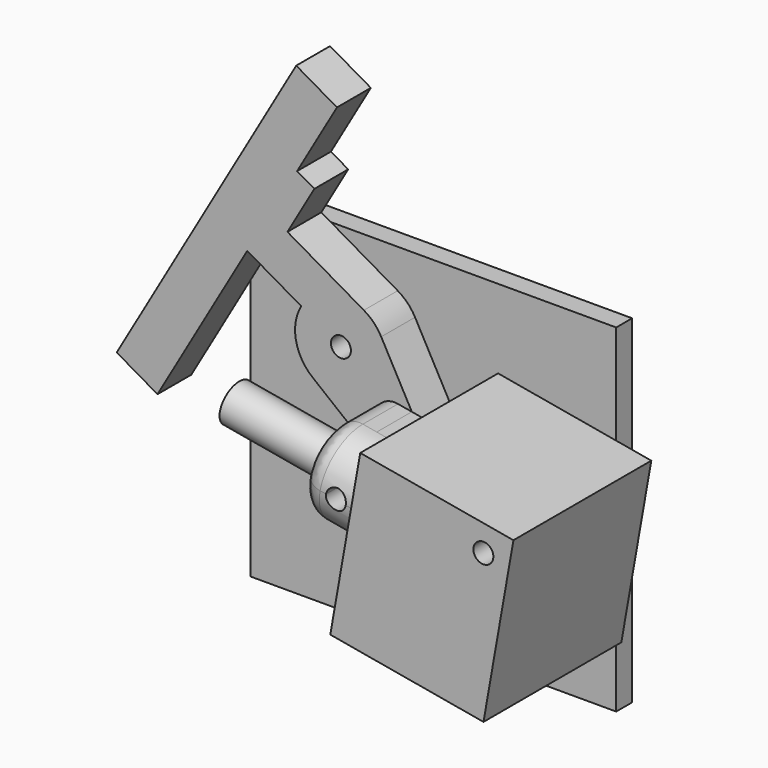
from build123d import *

# Parameters (mm, degrees)
F1_DEPTH    = 10.6
F2_DEPTH    = 43.2
F3_R        = 11
F4_DEPTH    = 2
F5_R        = 5
F6_DEPTH    = 43.4
F8_DEPTH    = 22
F9_T1_DEPTH = 73
F9_T3_DEPTH = 73
F10_W       = 91.6676837951
F10_H       = 84.7782492638
F11_DEPTH   = 5
F12_R       = 2.5
F13_DEPTH   = 74.8
F15_DEPTH   = 10.6
F16_R       = 5


# Not quite as in the source:
# - a fillet or chamfer that OpenCascade refuses, or shapes differently, is made with other operations: its cross-section is extruded or revolved along the edge and cut away or added
# - a feature names something its author has since deleted; it is built from what else it names


with BuildPart() as f1:
    # F0 (on Front) → F1 (new body)
    with BuildSketch(Plane.XZ):
        with BuildLine():
            Line((22.031131561, -16.3413353843), (10.0922695634, 5.5132653717))
            ThreePointArc((10.0922695634, 5.5132653717), (8.2271601871, 8.0351624287), (5.75, 9.9592921435))
            ThreePointArc((5.75, 9.9592921435), (-9.4974624505, 6.4844588827), (-7.1820107007, -8.9815768268))
            Line((-7.1820107007, -8.9815768268), (2.9745766929, -17.1031707017))
            Line((2.9745766929, -17.1031707017), (13.8647859035, -19.0234084111))
            ThreePointArc((13.8647859035, -19.0234084111), (16.5446946429, -16.96704211), (18.826805286, -19.4575288552))
            ThreePointArc((18.826805286, -19.4575288552), (18.8172920313, -19.6754182121), (18.7888246686, -19.8916492994))
            Line((18.7888246686, -19.8916492994), (22.7280556806, -20.5862420101))
            ThreePointArc((22.7280556806, -20.5862420101), (22.7409345871, -18.4044641332), (22.031131561, -16.3413353843))
        make_face()
        with BuildLine():
            ThreePointArc((2.5, 0), (-2.1650635095, -1.25), (1.25, 2.1650635095))
            ThreePointArc((1.25, 2.1650635095), (2.1650635095, 1.25), (2.5, 0))
        make_face(mode=Mode.SUBTRACT)
    extrude(amount=F1_DEPTH)

    # F14 (on face) → F15 (join)
    with BuildSketch(Plane.XZ.offset(10.6)):
        with BuildLine():
            Line((-17.7446848749, 23.5239547806), (-23.4946848749, 13.564662637))
            Line((-23.4946848749, 13.564662637), (-9.9592921435, 5.75))
            ThreePointArc((-9.9592921435, 5.75), (-2.9764190187, 11.1081470023), (5.75, 9.9592921435))
            Line((5.75, 9.9592921435), (-13.414557856, 21.0239547806))
            Line((-13.414557856, 21.0239547806), (-6.664557856, 32.7152977317))
            Line((-6.664557856, 32.7152977317), (-10.9946848749, 35.2152977317))
            Line((-10.9946848749, 35.2152977317), (-17.7446848749, 23.5239547806))
        make_face()
        Polygon((-41.6238499995, -4.8359724576), (-35.9946848749, -8.0859724576), (-23.4946848749, 13.564662637), (-17.7446848749, 23.5239547806), (-10.9946848749, 35.2152977317), (-16.6238499995, 38.4652977317), align=None)
        Polygon((-45.9946848749, -25.4064805333), (-35.9946848749, -8.0859724576), (-41.6238499995, -4.8359724576), (-16.6238499995, 38.4652977317), (-10.9946848749, 35.2152977317), (-0.9946848749, 52.5358058073), (-11.2137846395, 58.4358058073), (-56.2137846395, -19.5064805333), align=None)
    extrude(amount=-F15_DEPTH)


with BuildPart() as f1b:
    # F0 (on Front) → F1, piece 2 (new body)
    with BuildSketch(Plane.XZ):
        with BuildLine():
            ThreePointArc((12.2674079335, -24.5340722791), (17.833993936, -25.7803749211), (22.2397717789, -22.1569412458))
            Line((22.2397717789, -22.1569412458), (11.4577686407, -23.8866538829))
            Line((11.4577686407, -23.8866538829), (12.2674079335, -24.5340722791))
        make_face()
    extrude(amount=F1_DEPTH)


with BuildPart() as f2:
    # F0 (on Front) → F2 (new body)
    with BuildSketch(Plane.XZ):
        Polygon((30.9104912068, -0.0958113445), (27.1596905692, -21.3676588096), (23.4088899316, -42.6395062746), (61.816392299, -49.4117852036), (69.3179935743, -6.8680902735), align=None)
    extrude(amount=F2_DEPTH)

    # F3 (on face) → F4 (join)
    with BuildSketch(Plane(origin=(29.9948105542, 0, -5.2888943819), x_dir=(0, -1, 0), z_dir=(-0.984807753, 0, 0.1736481777))):
        with Locations((21.6, -16.326805286)):
            Circle(F3_R)
    extrude(amount=F4_DEPTH)

    # F5 (on face) → F6 (join)
    with BuildSketch(Plane(origin=(28.0251950482, 0, -4.9415980266), x_dir=(0, -1, 0), z_dir=(-0.984807753, 0, 0.1736481777))):
        with Locations((21.6, -16.326805286)):
            Circle(F5_R)
    extrude(amount=F6_DEPTH)


with BuildPart() as f8:
    # F7 (on face) → F8 (new body)
    with BuildSketch(Plane.XZ.offset(10.6)):
        with BuildLine():
            ThreePointArc((18.7888246686, -19.8916492994), (15.8926848419, -21.9195482378), (13.8647859035, -19.0234084111))
            Line((13.8647859035, -19.0234084111), (7.4635355089, -17.8946952562))
            Line((7.4635355089, -17.8946952562), (5.5534055546, -28.7275805394))
            Line((5.5534055546, -28.7275805394), (23.2799451088, -31.8532477374))
            Line((23.2799451088, -31.8532477374), (27.1002050175, -10.1874771711))
            Line((27.1002050175, -10.1874771711), (17.7707010183, -8.5424338994))
            Line((17.7707010183, -8.5424338994), (22.031131561, -16.3413353843))
            ThreePointArc((22.031131561, -16.3413353843), (22.7409345871, -18.4044641332), (22.7280556806, -20.5862420101))
            Line((22.7280556806, -20.5862420101), (18.7888246686, -19.8916492994))
        make_face()
        with BuildLine():
            ThreePointArc((13.8647859035, -19.0234084111), (16.5446946429, -16.96704211), (18.826805286, -19.4575288552))
            ThreePointArc((18.826805286, -19.4575288552), (18.8172920313, -19.6754182121), (18.7888246686, -19.8916492994))
            Line((18.7888246686, -19.8916492994), (22.7280556806, -20.5862420101))
            ThreePointArc((22.7280556806, -20.5862420101), (22.7409345871, -18.4044641332), (22.031131561, -16.3413353843))
            Line((22.031131561, -16.3413353843), (17.7707010183, -8.5424338994))
            Line((17.7707010183, -8.5424338994), (9.3736654633, -7.0618099731))
            Line((9.3736654633, -7.0618099731), (7.4635355089, -17.8946952562))
            Line((7.4635355089, -17.8946952562), (13.8647859035, -19.0234084111))
        make_face()
    extrude(amount=F8_DEPTH)

    # F9: fillet of radius 11 on 2 edges, made by hand

    # F9_s2 → F9_t1 (cut)
    with BuildSketch(Plane(origin=(55.107408256, 0, -9.7169229125), x_dir=(0, 1, 0), z_dir=(-0.984807753, 0, 0.1736481777))):
        with BuildLine():
            ThreePointArc((-21.6, 5.326805286), (-29.3781745931, 8.548630693), (-32.6, 16.326805286))
            Line((-32.6, 16.326805286), (-32.6, 5.326805286))
            Line((-32.6, 5.326805286), (-21.6, 5.326805286))
        make_face()
    extrude(amount=F9_T1_DEPTH, mode=Mode.SUBTRACT)

    # F9_s4 → F9_t3 (cut)
    with BuildSketch(Plane(origin=(-16.7835577139, 0, 2.9593940572), x_dir=(0, 1, 0), z_dir=(0.984807753, 0, -0.1736481777))):
        with BuildLine():
            ThreePointArc((-21.6, -27.326805286), (-29.3781745931, -24.1049798791), (-32.6, -16.326805286))
            Line((-32.6, -16.326805286), (-32.6, -27.326805286))
            Line((-32.6, -27.326805286), (-21.6, -27.326805286))
        make_face()
    extrude(amount=F9_T3_DEPTH, mode=Mode.SUBTRACT)

    # F16
    f16_edges = [f8.edges().sort_by_distance(p)[0] for p in [
        (8.814201, -29.378175, -10.234689),
        (5.553406, -16.1, -28.727581),
        (6.11287, -29.378175, -25.554702),
        (9.373665, -16.1, -7.06181),
    ]]
    fillet(f16_edges, radius=F16_R)


with BuildPart() as f11:
    # F10 (on face) → F11 (new body)
    with BuildSketch(Plane.XZ):
        with Locations((14.6878799424, -22.7255448699)):
            Rectangle(F10_W, F10_H)
        with BuildLine():
            Line((10.0922695634, 5.5132653717), (22.031131561, -16.3413353843))
            ThreePointArc((22.031131561, -16.3413353843), (22.7409345871, -18.4044641332), (22.7280556806, -20.5862420101))
            Line((22.7280556806, -20.5862420101), (18.7888246686, -19.8916492994))
            ThreePointArc((18.7888246686, -19.8916492994), (18.8172920313, -19.6754182121), (18.826805286, -19.4575288552))
            ThreePointArc((18.826805286, -19.4575288552), (16.5446946429, -16.96704211), (13.8647859035, -19.0234084111))
            Line((13.8647859035, -19.0234084111), (2.9745766929, -17.1031707017))
            Line((2.9745766929, -17.1031707017), (-7.1820107007, -8.9815768268))
            ThreePointArc((-7.1820107007, -8.9815768268), (-9.4974624505, 6.4844588827), (5.75, 9.9592921435))
            ThreePointArc((5.75, 9.9592921435), (8.2271601871, 8.0351624287), (10.0922695634, 5.5132653717))
        make_face(mode=Mode.SUBTRACT)
    extrude(amount=-F11_DEPTH)

    # F0 (on Front) → F11, piece 2 (join)
    with BuildSketch(Plane.XZ):
        with BuildLine():
            Line((22.031131561, -16.3413353843), (10.0922695634, 5.5132653717))
            ThreePointArc((10.0922695634, 5.5132653717), (8.2271601871, 8.0351624287), (5.75, 9.9592921435))
            ThreePointArc((5.75, 9.9592921435), (-9.4974624505, 6.4844588827), (-7.1820107007, -8.9815768268))
            Line((-7.1820107007, -8.9815768268), (2.9745766929, -17.1031707017))
            Line((2.9745766929, -17.1031707017), (13.8647859035, -19.0234084111))
            ThreePointArc((13.8647859035, -19.0234084111), (16.5446946429, -16.96704211), (18.826805286, -19.4575288552))
            ThreePointArc((18.826805286, -19.4575288552), (18.8172920313, -19.6754182121), (18.7888246686, -19.8916492994))
            Line((18.7888246686, -19.8916492994), (22.7280556806, -20.5862420101))
            ThreePointArc((22.7280556806, -20.5862420101), (22.7409345871, -18.4044641332), (22.031131561, -16.3413353843))
        make_face()
        with BuildLine():
            ThreePointArc((2.5, 0), (-2.1650635095, -1.25), (1.25, 2.1650635095))
            ThreePointArc((1.25, 2.1650635095), (2.1650635095, 1.25), (2.5, 0))
        make_face(mode=Mode.SUBTRACT)
        with BuildLine():
            ThreePointArc((13.8647859035, -19.0234084111), (15.8926848419, -21.9195482378), (18.7888246686, -19.8916492994))
            Line((18.7888246686, -19.8916492994), (13.8647859035, -19.0234084111))
        make_face()
        with BuildLine():
            Line((13.8647859035, -19.0234084111), (18.7888246686, -19.8916492994))
            ThreePointArc((18.7888246686, -19.8916492994), (18.8172920313, -19.6754182121), (18.826805286, -19.4575288552))
            ThreePointArc((18.826805286, -19.4575288552), (16.5446946429, -16.96704211), (13.8647859035, -19.0234084111))
        make_face()
    extrude(amount=-F11_DEPTH)


with BuildPart() as f13_tool:
    # F12 (on face) → F13 (new body)
    with BuildSketch(Plane.XZ.offset(43.2)):
        with Locations((61.7880300248, -12.1406275132)):
            Circle(F12_R)
    extrude(amount=-F13_DEPTH)


with BuildPart() as f2_1:
    add(f2.part)

    # F13: cut by f13_tool
    add(f13_tool.part, mode=Mode.SUBTRACT)


with BuildPart() as f11_1:
    add(f11.part)

    # F13: cut by f13_tool
    add(f13_tool.part, mode=Mode.SUBTRACT)


solid = Compound([f1.part, f1b.part, f8.part, f2_1.part, f11_1.part])
